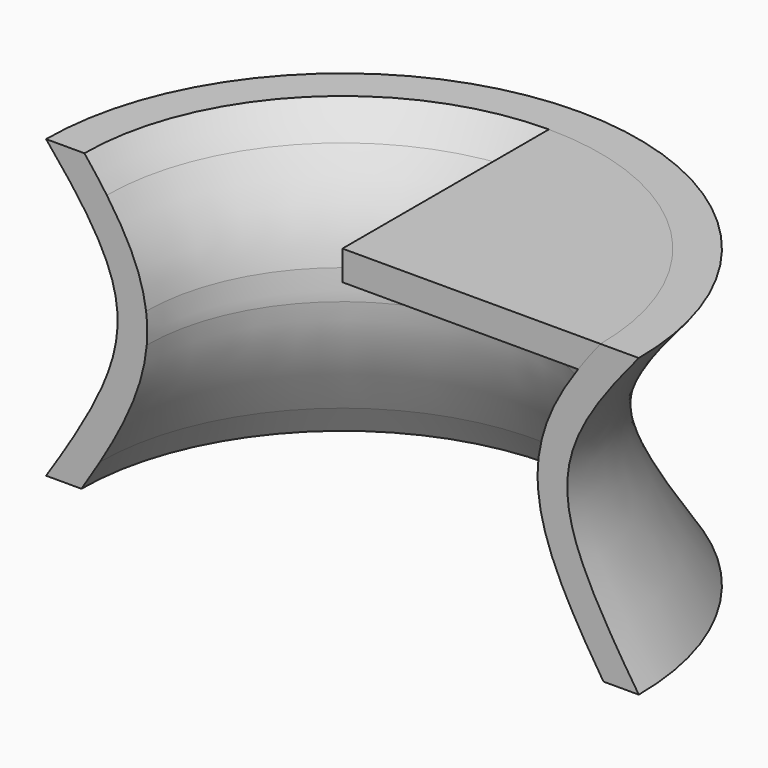
from build123d import *

# Parameters (mm, degrees)
F1_ANGLE = 180


# Not quite as in the source:
# - ends of sketch curves that miss each other by under 0.0002 mm in the source are joined
# - the dataset's text gives a spline's control points without its knots; the knots are read off the source's solid


with BuildPart() as f1:
    # F0 (on Front) → F1 (revolve)
    with BuildSketch(Plane.XZ):
        with BuildLine():
            Line((50, 50), (43.5300743603, 50))
            add(Edge.make_bspline(
                [(43.5300743603, 50), (42.498067868, 48.7104136359), (41.207824257, 47.0354225577), (40.0436420871, 45.4120413187), (39.7544855725, 45)],
                knots=[0.0558462552, 0.0558462552, 0.0558462552, 0.0558462552, 0.125, 0.1487334727, 0.1487334727, 0.1487334727, 0.1487334727], degree=3))
            add(Edge.make_bspline(
                [(39.7544855725, 45), (38.5207059056, 43.2418926245), (36.76988376, 40.4795697698), (34.9172349742, 36.6688421299), (33.7756100084, 33.4592340879), (33.2910956395, 31.1919070976), (33.1319464411, 30.0086565327), (33.1219467571, 29.9313710004)],
                knots=[0.1487334727, 0.1487334727, 0.1487334727, 0.1487334727, 0.25, 0.3125, 0.375, 0.4375, 0.4418647521, 0.4418647521, 0.4418647521, 0.4418647521], degree=3))
            add(Edge.make_bspline(
                [(33.1219467571, 29.9313710004), (32.9887584124, 28.9019852662), (32.8857676227, 27.2362651809), (32.9618442306, 25.5629192693), (33.0149946827, 24.9313798174)],
                knots=[0.4418647521, 0.4418647521, 0.4418647521, 0.4418647521, 0.5, 0.5351958944, 0.5351958944, 0.5351958944, 0.5351958944], degree=3))
            add(Edge.make_bspline(
                [(33.0149946827, 24.9313798174), (33.0562274906, 24.4414471094), (33.2402631381, 22.8290371112), (33.8138691799, 20.0937883976), (34.9227976374, 16.7039009591), (36.8929652729, 12.0841551613), (39.0229521213, 8.1686692531), (40.7598573349, 5.259995821), (40.9161858047, 5.0000254271)],
                knots=[0.5351958944, 0.5351958944, 0.5351958944, 0.5351958944, 0.5625, 0.625, 0.6875, 0.75, 0.875, 0.8871758141, 0.8871758141, 0.8871758141, 0.8871758141], degree=3))
            add(Edge.make_bspline(
                [(40.9161858047, 5.0000254271), (41.8745680412, 3.4062593792), (42.9141177909, 1.745043259), (44.0357419375, -1.3856e-05)],
                knots=[0.8871758141, 0.8871758141, 0.8871758141, 0.8871758141, 0.9618204647, 0.9618204647, 0.9618204647, 0.9618204647], degree=3))
            Line((44.0357419375, -1.3856e-05), (50, 0))
            add(Edge.make_bspline(
                [(50, 50), (33.761266619, 30.6610539556), (34.0517088771, 24.2713484913), (50, 0)],
                knots=[0, 0, 0, 0, 50, 50, 50, 50], degree=3))
        make_face()
    revolve(axis=Axis((0, 0, 25), (0, 0, 1)), revolution_arc=F1_ANGLE)


with BuildPart() as f2:
    # F0 (on Front) → F2 (new body, up to the next surface of F1)
    with BuildSketch(Plane.XZ):
        with BuildLine():
            Line((43.5300743603, 50), (0, 50))
            Line((0, 50), (0, 45))
            Line((0, 45), (39.7544855725, 45))
            add(Edge.make_bspline(
                [(43.5300743603, 50), (42.498067868, 48.7104136359), (41.207824257, 47.0354225577), (40.0436420871, 45.4120413187), (39.7544855725, 45)],
                knots=[0.0558462552, 0.0558462552, 0.0558462552, 0.0558462552, 0.125, 0.1487334727, 0.1487334727, 0.1487334727, 0.1487334727], degree=3))
        make_face()
    extrude(until=Until.NEXT, target=f1.part, dir=(0, 1, 0))


solid = Compound([f1.part, f2.part])
